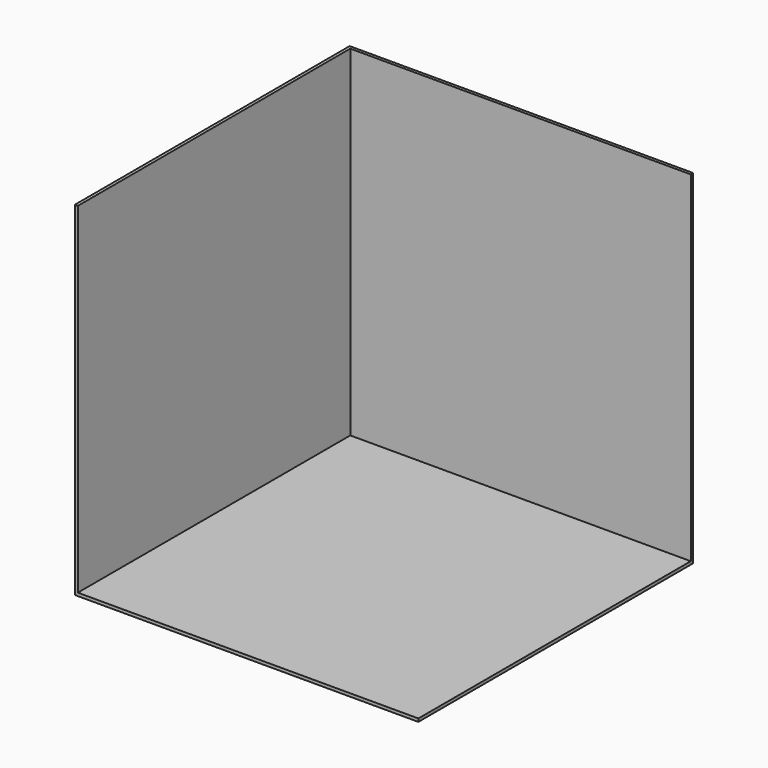
from build123d import *

# Parameters (mm, degrees)
F0_W     = 89.2000017881
F0_H     = 89.2
F1_DEPTH = 0.8
F2_DEPTH = 90


# Not quite as in the source:
# - ends of sketch curves that miss each other by under 0.0002 mm in the source are joined


with BuildPart() as f1:
    # F0 (on Top) → F1 (new body)
    with BuildSketch(Plane.XY):
        with Locations((0.3999991059, -0.4)):
            Rectangle(F0_W, F0_H)
    extrude(amount=F1_DEPTH)

    # F0 (on Top) → F2 (join)
    with BuildSketch(Plane.XY):
        Polygon((-45, -45), (-44.2000017881, -45), (-44.2000017881, 44.2), (-45.0000017881, 44.2), align=None)
        Polygon((-44.2000017881, 44.2), (44.9999982119, 44.2), (45, 45), (-45, 45), (-45, 44.2), align=None)
    extrude(amount=F2_DEPTH)


solid = f1.part
